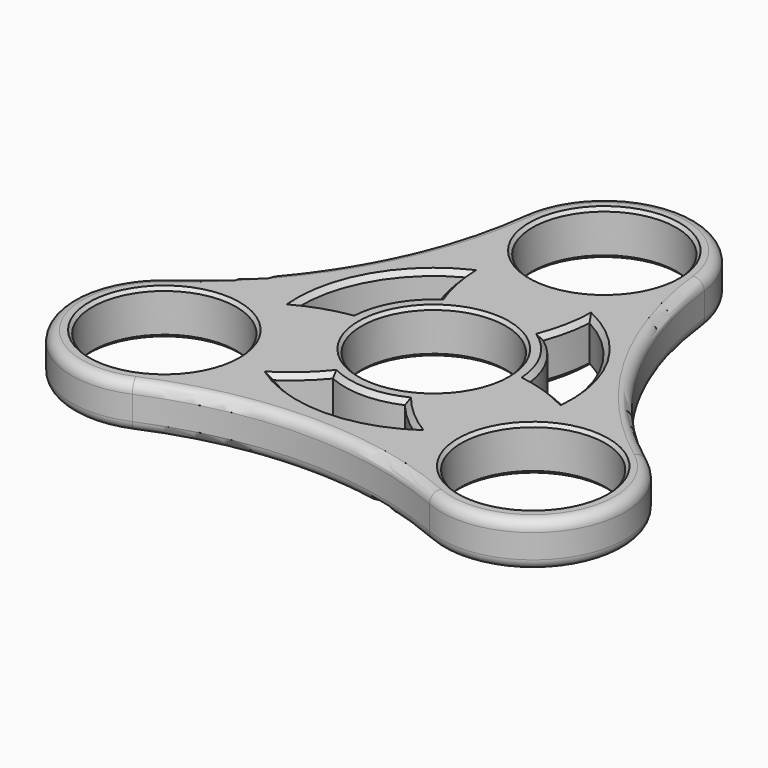
from build123d import *

# Parameters (mm, degrees)
F0_R          = 11.2522
F1_DEPTH      = 7
F2_R          = 11.2395
F3_DEPTH      = 7.001
F5_DEPTH      = 7.001
F6_R          = 1.625
F7_T3_ANGLE   = 75.0183506804
F7_S4_R       = 25.4
F7_T5_DEPTH   = 15
F7_S6_R       = 25.4
F7_T7_DEPTH   = 15
F7_T10_ANGLE  = 25.1712856634
F7_S11_R      = 13.843
F7_T12_DEPTH  = 7
F7_S13_R      = 20.701
F7_T14_DEPTH  = 7
F7_T17_ANGLE  = 63.8377846637
F7_S18_R      = 25.4
F7_T19_DEPTH  = 9
F7_S20_R      = 25.4
F7_T21_DEPTH  = 9
F7_T24_ANGLE  = 25.1712856634
F7_S25_R      = 13.843
F7_T26_DEPTH  = 7
F7_S27_R      = 20.701
F7_T28_DEPTH  = 7
F7_T31_ANGLE  = 25.1712856634
F7_S32_R      = 20.701
F7_T33_DEPTH  = 7
F7_S34_R      = 13.843
F7_T35_DEPTH  = 7
F7_T38_ANGLE  = 63.8377846637
F7_S39_R      = 25.4
F7_T40_DEPTH  = 9
F7_S41_R      = 25.4
F7_T42_DEPTH  = 9
F7_T45_ANGLE  = 25.1712856634
F7_S46_R      = 20.701
F7_T47_DEPTH  = 7
F7_S48_R      = 13.843
F7_T49_DEPTH  = 7
F7_T52_ANGLE  = 75.0183506804
F7_S53_R      = 25.4
F7_T54_DEPTH  = 15
F7_S55_R      = 25.4
F7_T56_DEPTH  = 15
F7_T59_ANGLE  = 25.1712856634
F7_S60_R      = 20.701
F7_T61_DEPTH  = 7
F7_S62_R      = 13.843
F7_T63_DEPTH  = 7
F7_T66_ANGLE  = 63.8377846637
F7_S67_R      = 25.4
F7_T68_DEPTH  = 9
F7_S69_R      = 25.4
F7_T70_DEPTH  = 9
F7_T73_ANGLE  = 25.1712856634
F7_S74_R      = 20.701
F7_T75_DEPTH  = 7
F7_S76_R      = 13.843
F7_T77_DEPTH  = 7
F7_T80_ANGLE  = 75.0183506804
F7_S81_R      = 25.4
F7_T82_DEPTH  = 15
F7_S83_R      = 25.4
F7_T84_DEPTH  = 15
F7_T87_ANGLE  = 75.0183506804
F7_S88_R      = 25.4
F7_T89_DEPTH  = 15
F7_S90_R      = 25.4
F7_T91_DEPTH  = 15
F7_T94_ANGLE  = 63.8377846637
F7_S95_R      = 25.4
F7_T96_DEPTH  = 9
F7_S97_R      = 25.4
F7_T98_DEPTH  = 9
F7_T101_ANGLE = 25.1712856634
F7_S102_R     = 20.701
F7_T103_DEPTH = 7
F7_S104_R     = 13.843
F7_T105_DEPTH = 7
F7_T108_ANGLE = 25.1712856634
F7_S109_R     = 20.701
F7_T110_DEPTH = 7
F7_S111_R     = 13.843
F7_T112_DEPTH = 7
F7_T115_ANGLE = 25.1712856634
F7_S116_R     = 20.701
F7_T117_DEPTH = 7
F7_S118_R     = 13.843
F7_T119_DEPTH = 7
F7_T122_ANGLE = 75.0183506804
F7_S123_R     = 25.4
F7_T124_DEPTH = 15
F7_S125_R     = 25.4
F7_T126_DEPTH = 15
F7_T129_ANGLE = 63.8377846637
F7_S130_R     = 25.4
F7_T131_DEPTH = 9
F7_S132_R     = 25.4
F7_T133_DEPTH = 9
F7_T136_ANGLE = 25.1712856634
F7_S137_R     = 20.701
F7_T138_DEPTH = 7
F7_S139_R     = 13.843
F7_T140_DEPTH = 7
F7_T143_ANGLE = 25.1712856634
F7_S144_R     = 13.843
F7_T145_DEPTH = 7
F7_S146_R     = 20.701
F7_T147_DEPTH = 7
F7_T150_ANGLE = 75.0183506804
F7_S151_R     = 25.4
F7_T152_DEPTH = 15
F7_S153_R     = 25.4
F7_T154_DEPTH = 15
F7_T157_ANGLE = 25.1712856634
F7_S158_R     = 13.843
F7_T159_DEPTH = 7
F7_S160_R     = 20.701
F7_T161_DEPTH = 7
F7_T164_ANGLE = 63.8377846637
F7_S165_R     = 25.4
F7_T166_DEPTH = 9
F7_S167_R     = 25.4
F7_T168_DEPTH = 9
F7_T172_ANGLE = 25.1712856634
F7_S173_R     = 20.701
F7_T174_DEPTH = 7
F7_T177_ANGLE = 75.0183506804
F7_S178_R     = 25.4
F7_T179_DEPTH = 15
F7_T184_ANGLE = 25.1712856634
F7_S185_R     = 20.701
F7_T186_DEPTH = 7
F7_T189_ANGLE = 75.0183506804
F7_S190_R     = 25.4
F7_T191_DEPTH = 15
F7_T196_ANGLE = 63.8377846637
F7_S197_R     = 25.4
F7_T198_DEPTH = 9
F7_T201_ANGLE = 25.1712856634
F7_S202_R     = 13.843
F7_T203_DEPTH = 7
F7_T208_ANGLE = 25.1712856634
F7_S209_R     = 13.843
F7_T210_DEPTH = 7
F7_T213_ANGLE = 63.8377846637
F7_S214_R     = 25.4
F7_T215_DEPTH = 9
F7_T220_ANGLE = 75.0183506804
F7_S221_R     = 25.4
F7_T222_DEPTH = 15
F7_T225_ANGLE = 25.1712856634
F7_S226_R     = 20.701
F7_T227_DEPTH = 7
F7_T232_ANGLE = 25.1712856634
F7_S233_R     = 13.843
F7_T234_DEPTH = 7
F7_T237_ANGLE = 63.8377846637
F7_S238_R     = 25.4
F7_T239_DEPTH = 9
F7_T244_ANGLE = 25.1712856634
F7_S245_R     = 13.843
F7_T246_DEPTH = 7
F7_T249_ANGLE = 63.8377846637
F7_S250_R     = 25.4
F7_T251_DEPTH = 9
F7_T256_ANGLE = 25.1712856634
F7_S257_R     = 20.701
F7_T258_DEPTH = 7
F7_T261_ANGLE = 75.0183506804
F7_S262_R     = 25.4
F7_T263_DEPTH = 15
F7_T268_ANGLE = 75.0183506804
F7_S269_R     = 25.4
F7_T270_DEPTH = 15
F7_T273_ANGLE = 25.1712856634
F7_S274_R     = 20.701
F7_T275_DEPTH = 7
F7_T280_ANGLE = 25.1712856634
F7_S281_R     = 13.843
F7_T282_DEPTH = 7
F7_T285_ANGLE = 63.8377846637
F7_S286_R     = 25.4
F7_T287_DEPTH = 9
F7_T292_ANGLE = 25.1712856634
F7_S293_R     = 13.843
F7_T294_DEPTH = 7
F7_T297_ANGLE = 63.8377846637
F7_S298_R     = 25.4
F7_T299_DEPTH = 9
F7_T304_ANGLE = 25.1712856634
F7_S305_R     = 20.701
F7_T306_DEPTH = 7
F7_T309_ANGLE = 75.0183506804
F7_S310_R     = 25.4
F7_T311_DEPTH = 15
F7_T316_ANGLE = 75.0183506804
F7_S317_R     = 25.4
F7_T318_DEPTH = 15
F7_T321_ANGLE = 25.1712856634
F7_S322_R     = 20.701
F7_T323_DEPTH = 7
F7_T328_ANGLE = 75.0183506804
F7_S329_R     = 25.4
F7_T330_DEPTH = 15
F7_T333_ANGLE = 25.1712856634
F7_S334_R     = 20.701
F7_T335_DEPTH = 7
F7_T340_ANGLE = 63.8377846637
F7_S341_R     = 25.4
F7_T342_DEPTH = 9
F7_T345_ANGLE = 25.1712856634
F7_S346_R     = 13.843
F7_T347_DEPTH = 7
F7_T352_ANGLE = 25.1712856634
F7_S353_R     = 13.843
F7_T354_DEPTH = 7
F7_T357_ANGLE = 63.8377846637
F7_S358_R     = 25.4
F7_T359_DEPTH = 9
F7_T364_ANGLE = 75.0183506804
F7_S365_R     = 25.4
F7_T366_DEPTH = 15
F7_T369_ANGLE = 25.1712856634
F7_S370_R     = 20.701
F7_T371_DEPTH = 7
F7_T376_ANGLE = 63.8377846637
F7_S377_R     = 25.4
F7_T378_DEPTH = 9
F7_T381_ANGLE = 25.1712856634
F7_S382_R     = 13.843
F7_T383_DEPTH = 7
F7_T388_ANGLE = 75.0183506804
F7_S389_R     = 25.4
F7_T390_DEPTH = 15
F7_T393_ANGLE = 25.1712856634
F7_S394_R     = 20.701
F7_T395_DEPTH = 7
F7_T400_ANGLE = 25.1712856634
F7_S401_R     = 13.843
F7_T402_DEPTH = 7
F7_T405_ANGLE = 63.8377846637
F7_S406_R     = 25.4
F7_T407_DEPTH = 9
F7_T412_ANGLE = 25.1712856634
F7_S413_R     = 20.701
F7_T414_DEPTH = 7
F7_T417_ANGLE = 75.0183506804
F7_S418_R     = 25.4
F7_T419_DEPTH = 15
F7_T424_ANGLE = 63.8377846637
F7_S425_R     = 25.4
F7_T426_DEPTH = 9
F7_T429_ANGLE = 25.1712856634
F7_S430_R     = 13.843
F7_T431_DEPTH = 7
F7_T436_ANGLE = 75.0183506804
F7_S437_R     = 25.4
F7_T438_DEPTH = 15
F7_T441_ANGLE = 25.1712856634
F7_S442_R     = 20.701
F7_T443_DEPTH = 7
F7_T448_ANGLE = 63.8377846637
F7_S449_R     = 25.4
F7_T450_DEPTH = 9
F7_T453_ANGLE = 25.1712856634
F7_S454_R     = 13.843
F7_T455_DEPTH = 7
F8_SIZE       = 0.5


# Not quite as in the source:
# - a fillet or chamfer that OpenCascade refuses, or shapes differently, is made with other operations: its cross-section is extruded or revolved along the edge and cut away or added


with BuildPart() as f1:
    # F0 (on Top) → F1 (new body)
    with BuildSketch(Plane.XY):
        with BuildLine():
            ThreePointArc((37.4145413955, -5.1495366448), (21.713132902, 12.5325990694), (14.2502695702, 34.9713562316))
            ThreePointArc((14.2502695702, 34.9713562316), (-0.0001243489, 47.6249999995), (-14.2502989826, 34.9711092792))
            ThreePointArc((-14.2502989826, 34.9711092792), (-21.7127734575, 12.5322227915), (-37.4138755234, -5.1501850199))
            ThreePointArc((-37.4138755234, -5.1501850199), (-41.2470555173, -23.8182100517), (-23.1633773799, -29.8322779327))
            ThreePointArc((-23.1633773799, -29.8322779327), (0.0005055885, -25.0755271592), (23.1644709862, -29.83187651))
            ThreePointArc((23.1644709862, -29.83187651), (41.2480448991, -23.8174952461), (37.4145413955, -5.1495366448))
        make_face()
        Circle(F0_R, mode=Mode.SUBTRACT)
    extrude(amount=F1_DEPTH)

    # F2 (on face) → F3 (cut, through all)
    with BuildSketch(Plane.XY.offset(7)):
        with Locations((0, 33.274)):
            Circle(F2_R)
        with Locations((-28.7836054376, -16.5806670429)):
            Circle(F2_R)
        with Locations((28.7836054376, -16.5806670429)):
            Circle(F2_R)
    extrude(amount=-F3_DEPTH, mode=Mode.SUBTRACT)

    # F4 (on face) → F5 (cut, through all)
    with BuildSketch(Plane.XY.offset(7)):
        with BuildLine():
            ThreePointArc((5.6160809719, -12.6525998718), (-6.831e-07, -13.843), (-5.6160822206, -12.6525993176))
            ThreePointArc((-5.6160822206, -12.6525993176), (-8.1436475782, -15.2823065658), (-11.021805406, -17.5228766643))
            ThreePointArc((-11.021805406, -17.5228766643), (-1.0215e-06, -20.701), (11.0218036767, -17.522877752))
            ThreePointArc((11.0218036767, -17.522877752), (8.14364607, -15.2823073695), (5.6160809719, -12.6525998718))
        make_face()
        with BuildLine():
            ThreePointArc((-8.1494313227, 11.1899695315), (-9.1630419253, 14.6937589651), (-9.6643536357, 18.3066018093))
            ThreePointArc((-9.6643536357, 18.3066018093), (-17.927591373, 10.3505008846), (-20.686159119, -0.7837231035))
            ThreePointArc((-20.686159119, -0.7837231035), (-17.3066894454, 0.5885493087), (-13.7655133989, 1.4626311446))
            ThreePointArc((-13.7655133989, 1.4626311446), (-11.9883893231, 6.9215005916), (-8.1494313227, 11.1899695315))
        make_face()
        with BuildLine():
            ThreePointArc((9.6643554423, 18.3066008556), (9.1630433754, 14.6937580608), (8.149432427, 11.1899687273))
            ThreePointArc((8.149432427, 11.1899687273), (11.9883900061, 6.9214994084), (13.7655135432, 1.4626297861))
            ThreePointArc((13.7655135432, 1.4626297861), (17.3066895035, 0.5885476007), (20.6861590417, -0.783725145))
            ThreePointArc((20.6861590417, -0.783725145), (17.9275923945, 10.3504991154), (9.6643554423, 18.3066008556))
        make_face()
    extrude(amount=-F5_DEPTH, mode=Mode.SUBTRACT)

    # F6
    f6_edges = [f1.edges().sort_by_distance(p)[0] for p in [
        (0.000506, -25.075527, 7),
        (0.000506, -25.075527, 0),
        (41.248045, -23.817495, 0),
        (41.248045, -23.817495, 7),
        (21.713133, 12.532599, 0),
        (21.713133, 12.532599, 7),
        (-41.247056, -23.81821, 0),
        (-0.000124, 47.625, 0),
        (-21.712773, 12.532223, 0),
        (-41.247056, -23.81821, 7),
        (-0.000124, 47.625, 7),
        (-21.712773, 12.532223, 7),
    ]]
    fillet(f6_edges, radius=F6_R)

    # F7: chamfer of 0.75 on 24 edges, made by hand


with BuildPart() as f7_tool1:
    # F7_s2 → F7_t3 (revolve)
    with BuildSketch(Plane(origin=(0, 0, 0), x_dir=(0, 0, 1), z_dir=(0.9239408224, 0.3825354319, 0))):
        Polygon((7, -21.451), (6.25, -20.701), (7, -20.701), align=None)
    revolve(axis=Axis((0, 0, 7), (0, 0, 1)), revolution_arc=F7_T3_ANGLE)

    # F7_s4 → F7_t5 (cut, symmetric)
    with BuildSketch(Plane.XY.offset(6.6)):
        with Locations((15.6803190028, 19.9821819622)):
            Circle(F7_S4_R)
    extrude(amount=F7_T5_DEPTH, both=True, mode=Mode.SUBTRACT)

    # F7_s6 → F7_t7 (cut, symmetric)
    with BuildSketch(Plane.XY.offset(6.6)):
        with Locations((-9.4649200271, -23.5706446429)):
            Circle(F7_S6_R)
    extrude(amount=F7_T7_DEPTH, both=True, mode=Mode.SUBTRACT)


with BuildPart() as f7_tool8:
    # F7_s9 → F7_t10 (revolve)
    with BuildSketch(Plane(origin=(-4.8460279311, 10.583246727, 0), x_dir=(0, 0, 1), z_dir=(0.4163261949, -0.9092153207, 0))):
        Polygon((7, 2.0741079466), (6.25, 2.8241079466), (7, 2.8241079466), align=None)
    revolve(axis=Axis((15.6803190028, 19.9821819622, 7), (0, 0, -1)), revolution_arc=F7_T10_ANGLE)

    # F7_s11 → F7_t12 (cut, symmetric)
    with BuildSketch(Plane.XY.offset(6.6)):
        Circle(F7_S11_R)
    extrude(amount=F7_T12_DEPTH, both=True, mode=Mode.SUBTRACT)

    # F7_s13 → F7_t14 (intersect, symmetric)
    with BuildSketch(Plane.XY.offset(6.6)):
        Circle(F7_S13_R)
    extrude(amount=F7_T14_DEPTH, both=True, mode=Mode.INTERSECT)


with BuildPart() as f7_tool15:
    # F7_s16 → F7_t17 (revolve)
    with BuildSketch(Plane(origin=(0, 0, 0), x_dir=(0, 0, 1), z_dir=(0.0334846794, -0.9994392309, 0))):
        Polygon((7, 13.093), (6.25, 13.843), (7, 13.843), align=None)
    revolve(axis=Axis((0, 0, 7), (0, 0, -1)), revolution_arc=F7_T17_ANGLE)

    # F7_s18 → F7_t19 (cut, symmetric)
    with BuildSketch(Plane.XY.offset(6.6)):
        with Locations((15.6803190028, 19.9821819622)):
            Circle(F7_S18_R)
    extrude(amount=F7_T19_DEPTH, both=True, mode=Mode.SUBTRACT)

    # F7_s20 → F7_t21 (cut, symmetric)
    with BuildSketch(Plane.XY.offset(6.6)):
        with Locations((-9.4649200271, -23.5706446429)):
            Circle(F7_S20_R)
    extrude(amount=F7_T21_DEPTH, both=True, mode=Mode.SUBTRACT)


with BuildPart() as f7_tool22:
    # F7_s23 → F7_t24 (revolve)
    with BuildSketch(Plane(origin=(-17.3382017848, -10.2408889637, 0), x_dir=(0, 0, 1), z_dir=(-0.8610224768, -0.5085669027, 0))):
        Polygon((7, 9.1686902329), (6.25, 9.9186902329), (7, 9.9186902329), align=None)
    revolve(axis=Axis((-9.4649200271, -23.5706446429, 7), (0, 0, -1)), revolution_arc=F7_T24_ANGLE)

    # F7_s25 → F7_t26 (cut, symmetric)
    with BuildSketch(Plane.XY.offset(6.6)):
        Circle(F7_S25_R)
    extrude(amount=F7_T26_DEPTH, both=True, mode=Mode.SUBTRACT)

    # F7_s27 → F7_t28 (intersect, symmetric)
    with BuildSketch(Plane.XY.offset(6.6)):
        Circle(F7_S27_R)
    extrude(amount=F7_T28_DEPTH, both=True, mode=Mode.INTERSECT)


with BuildPart() as f7_tool29:
    # F7_s30 → F7_t31 (revolve)
    with BuildSketch(Plane(origin=(-0.1997691075, 20.1357676834, 0), x_dir=(0, 0, 1), z_dir=(-0.0099206189, 0.9999507894, 0))):
        Polygon((7, 9.1686902329), (6.25, 9.9186902329), (7, 9.9186902329), align=None)
    revolve(axis=Axis((-15.6803170308, 19.9821835097, 7), (0, 0, -1)), revolution_arc=F7_T31_ANGLE)

    # F7_s32 → F7_t33 (intersect, symmetric)
    with BuildSketch(Plane.XY.offset(6.6)):
        Circle(F7_S32_R)
    extrude(amount=F7_T33_DEPTH, both=True, mode=Mode.INTERSECT)

    # F7_s34 → F7_t35 (cut, symmetric)
    with BuildSketch(Plane.XY.offset(6.6)):
        Circle(F7_S34_R)
    extrude(amount=F7_T35_DEPTH, both=True, mode=Mode.SUBTRACT)


with BuildPart() as f7_tool36:
    # F7_s37 → F7_t38 (revolve)
    with BuildSketch(Plane(origin=(0, 0, 0), x_dir=(0, 0, 1), z_dir=(-0.8822821032, 0.4707210325, 0))):
        Polygon((7, 13.093), (6.25, 13.843), (7, 13.843), align=None)
    revolve(axis=Axis((0, 0, 7), (0, 0, -1)), revolution_arc=F7_T38_ANGLE)

    # F7_s39 → F7_t40 (cut, symmetric)
    with BuildSketch(Plane.XY.offset(6.6)):
        with Locations((-15.6803170308, 19.9821835097)):
            Circle(F7_S39_R)
    extrude(amount=F7_T40_DEPTH, both=True, mode=Mode.SUBTRACT)

    # F7_s41 → F7_t42 (cut, symmetric)
    with BuildSketch(Plane.XY.offset(6.6)):
        with Locations((9.4649177009, -23.570645577)):
            Circle(F7_S41_R)
    extrude(amount=F7_T42_DEPTH, both=True, mode=Mode.SUBTRACT)


with BuildPart() as f7_tool43:
    # F7_s44 → F7_t45 (revolve)
    with BuildSketch(Plane(origin=(11.5883744856, -1.0948400677, 0), x_dir=(0, 0, 1), z_dir=(-0.9955666627, 0.0940585993, 0))):
        Polygon((7, 2.0741079466), (6.25, 2.8241079466), (7, 2.8241079466), align=None)
    revolve(axis=Axis((9.4649177009, -23.570645577, 7), (0, 0, -1)), revolution_arc=F7_T45_ANGLE)

    # F7_s46 → F7_t47 (intersect, symmetric)
    with BuildSketch(Plane.XY.offset(6.6)):
        Circle(F7_S46_R)
    extrude(amount=F7_T47_DEPTH, both=True, mode=Mode.INTERSECT)

    # F7_s48 → F7_t49 (cut, symmetric)
    with BuildSketch(Plane.XY.offset(6.6)):
        Circle(F7_S48_R)
    extrude(amount=F7_T49_DEPTH, both=True, mode=Mode.SUBTRACT)


with BuildPart() as f7_tool50:
    # F7_s51 → F7_t52 (revolve)
    with BuildSketch(Plane(origin=(0, 0, 0), x_dir=(0, 0, 1), z_dir=(-0.1306850093, -0.9914239398, 0))):
        Polygon((7, -21.451), (6.25, -20.701), (7, -20.701), align=None)
    revolve(axis=Axis((0, 0, 7), (0, 0, 1)), revolution_arc=F7_T52_ANGLE)

    # F7_s53 → F7_t54 (cut, symmetric)
    with BuildSketch(Plane.XY.offset(6.6)):
        with Locations((-15.6803170308, 19.9821835097)):
            Circle(F7_S53_R)
    extrude(amount=F7_T54_DEPTH, both=True, mode=Mode.SUBTRACT)

    # F7_s55 → F7_t56 (cut, symmetric)
    with BuildSketch(Plane.XY.offset(6.6)):
        with Locations((9.4649177009, -23.570645577)):
            Circle(F7_S55_R)
    extrude(amount=F7_T56_DEPTH, both=True, mode=Mode.SUBTRACT)


with BuildPart() as f7_tool57:
    # F7_s58 → F7_t59 (revolve)
    with BuildSketch(Plane(origin=(17.5379708923, -9.8948787197, 0), x_dir=(0, 0, 1), z_dir=(0.8709430956, -0.4913838868, 0))):
        Polygon((7, 9.1686902329), (6.25, 9.9186902329), (7, 9.9186902329), align=None)
    revolve(axis=Axis((25.1452370578, 3.5884611332, 7), (0, 0, -1)), revolution_arc=F7_T59_ANGLE)

    # F7_s60 → F7_t61 (intersect, symmetric)
    with BuildSketch(Plane.XY.offset(6.6)):
        Circle(F7_S60_R)
    extrude(amount=F7_T61_DEPTH, both=True, mode=Mode.INTERSECT)

    # F7_s62 → F7_t63 (cut, symmetric)
    with BuildSketch(Plane.XY.offset(6.6)):
        Circle(F7_S62_R)
    extrude(amount=F7_T63_DEPTH, both=True, mode=Mode.SUBTRACT)


with BuildPart() as f7_tool64:
    # F7_s65 → F7_t66 (revolve)
    with BuildSketch(Plane(origin=(0, 0, 0), x_dir=(0, 0, 1), z_dir=(0.8487974238, 0.5287181984, 0))):
        Polygon((7, 13.093), (6.25, 13.843), (7, 13.843), align=None)
    revolve(axis=Axis((0, 0, 7), (0, 0, -1)), revolution_arc=F7_T66_ANGLE)

    # F7_s67 → F7_t68 (cut, symmetric)
    with BuildSketch(Plane.XY.offset(6.6)):
        with Locations((25.1452370578, 3.5884611332)):
            Circle(F7_S67_R)
    extrude(amount=F7_T68_DEPTH, both=True, mode=Mode.SUBTRACT)

    # F7_s69 → F7_t70 (cut, symmetric)
    with BuildSketch(Plane.XY.offset(6.6)):
        with Locations((-25.1452367037, 3.5884636148)):
            Circle(F7_S69_R)
    extrude(amount=F7_T70_DEPTH, both=True, mode=Mode.SUBTRACT)


with BuildPart() as f7_tool71:
    # F7_s72 → F7_t73 (revolve)
    with BuildSketch(Plane(origin=(-6.7423465545, -9.4884066593, 0), x_dir=(0, 0, 1), z_dir=(0.5792404678, 0.8151567214, 0))):
        Polygon((7, 2.0741079466), (6.25, 2.8241079466), (7, 2.8241079466), align=None)
    revolve(axis=Axis((-25.1452367037, 3.5884636148, 7), (0, 0, -1)), revolution_arc=F7_T73_ANGLE)

    # F7_s74 → F7_t75 (intersect, symmetric)
    with BuildSketch(Plane.XY.offset(6.6)):
        Circle(F7_S74_R)
    extrude(amount=F7_T75_DEPTH, both=True, mode=Mode.INTERSECT)

    # F7_s76 → F7_t77 (cut, symmetric)
    with BuildSketch(Plane.XY.offset(6.6)):
        Circle(F7_S76_R)
    extrude(amount=F7_T77_DEPTH, both=True, mode=Mode.SUBTRACT)


with BuildPart() as f7_tool78:
    # F7_s79 → F7_t80 (revolve)
    with BuildSketch(Plane(origin=(0, 0, 0), x_dir=(0, 0, 1), z_dir=(-0.7932558131, 0.6088885079, 0))):
        Polygon((7, -21.451), (6.25, -20.701), (7, -20.701), align=None)
    revolve(axis=Axis((0, 0, 7), (0, 0, 1)), revolution_arc=F7_T80_ANGLE)

    # F7_s81 → F7_t82 (cut, symmetric)
    with BuildSketch(Plane.XY.offset(6.6)):
        with Locations((25.1452370578, 3.5884611332)):
            Circle(F7_S81_R)
    extrude(amount=F7_T82_DEPTH, both=True, mode=Mode.SUBTRACT)

    # F7_s83 → F7_t84 (cut, symmetric)
    with BuildSketch(Plane.XY.offset(6.6)):
        with Locations((-25.1452367037, 3.5884636148)):
            Circle(F7_S83_R)
    extrude(amount=F7_T84_DEPTH, both=True, mode=Mode.SUBTRACT)


with BuildPart() as f7_tool85:
    # F7_s86 → F7_t87 (revolve)
    with BuildSketch(Plane(origin=(0, 0, 0), x_dir=(0, 0, 1), z_dir=(-0.7932558131, 0.6088885079, 0))):
        Polygon((0, -21.451), (0.75, -20.701), (0, -20.701), align=None)
    revolve(axis=Axis((0, 0, 0), (0, 0, 1)), revolution_arc=F7_T87_ANGLE)

    # F7_s88 → F7_t89 (cut, symmetric)
    with BuildSketch(Plane.XY.offset(0.4)):
        with Locations((25.1452370578, 3.5884611332)):
            Circle(F7_S88_R)
    extrude(amount=F7_T89_DEPTH, both=True, mode=Mode.SUBTRACT)

    # F7_s90 → F7_t91 (cut, symmetric)
    with BuildSketch(Plane.XY.offset(0.4)):
        with Locations((-25.1452367037, 3.5884636148)):
            Circle(F7_S90_R)
    extrude(amount=F7_T91_DEPTH, both=True, mode=Mode.SUBTRACT)


with BuildPart() as f7_tool92:
    # F7_s93 → F7_t94 (revolve)
    with BuildSketch(Plane(origin=(0, 0, 0), x_dir=(0, 0, 1), z_dir=(-0.8487973716, 0.5287182822, 0))):
        Polygon((0, -13.093), (0.75, -13.843), (0, -13.843), align=None)
    revolve(axis=Axis((0, 0, 0), (0, 0, 1)), revolution_arc=F7_T94_ANGLE)

    # F7_s95 → F7_t96 (cut, symmetric)
    with BuildSketch(Plane.XY.offset(0.4)):
        with Locations((25.1452370578, 3.5884611332)):
            Circle(F7_S95_R)
    extrude(amount=F7_T96_DEPTH, both=True, mode=Mode.SUBTRACT)

    # F7_s97 → F7_t98 (cut, symmetric)
    with BuildSketch(Plane.XY.offset(0.4)):
        with Locations((-25.1452367037, 3.5884636148)):
            Circle(F7_S97_R)
    extrude(amount=F7_T98_DEPTH, both=True, mode=Mode.SUBTRACT)


with BuildPart() as f7_tool99:
    # F7_s100 → F7_t101 (revolve)
    with BuildSketch(Plane(origin=(-17.5379718688, -9.8948769889, 0), x_dir=(0, 0, 1), z_dir=(-0.8709431441, -0.4913838008, 0))):
        Polygon((0, -9.1686902329), (0.75, -9.9186902329), (0, -9.9186902329), align=None)
    revolve(axis=Axis((-25.1452367037, 3.5884636148, 0), (0, 0, 1)), revolution_arc=F7_T101_ANGLE)

    # F7_s102 → F7_t103 (intersect, symmetric)
    with BuildSketch(Plane.XY.offset(0.4)):
        Circle(F7_S102_R)
    extrude(amount=F7_T103_DEPTH, both=True, mode=Mode.INTERSECT)

    # F7_s104 → F7_t105 (cut, symmetric)
    with BuildSketch(Plane.XY.offset(0.4)):
        Circle(F7_S104_R)
    extrude(amount=F7_T105_DEPTH, both=True, mode=Mode.SUBTRACT)


with BuildPart() as f7_tool106:
    # F7_s107 → F7_t108 (revolve)
    with BuildSketch(Plane(origin=(6.7423456181, -9.4884073247, 0), x_dir=(0, 0, 1), z_dir=(-0.5792403874, 0.8151567786, 0))):
        Polygon((0, -2.0741079466), (0.75, -2.8241079466), (0, -2.8241079466), align=None)
    revolve(axis=Axis((25.1452370578, 3.5884611332, 0), (0, 0, 1)), revolution_arc=F7_T108_ANGLE)

    # F7_s109 → F7_t110 (intersect, symmetric)
    with BuildSketch(Plane.XY.offset(0.4)):
        Circle(F7_S109_R)
    extrude(amount=F7_T110_DEPTH, both=True, mode=Mode.INTERSECT)

    # F7_s111 → F7_t112 (cut, symmetric)
    with BuildSketch(Plane.XY.offset(0.4)):
        Circle(F7_S111_R)
    extrude(amount=F7_T112_DEPTH, both=True, mode=Mode.SUBTRACT)


with BuildPart() as f7_tool113:
    # F7_s114 → F7_t115 (revolve)
    with BuildSketch(Plane(origin=(17.3382007741, -10.2408906747, 0), x_dir=(0, 0, 1), z_dir=(0.8610224266, -0.5085669877, 0))):
        Polygon((0, -9.1686902329), (0.75, -9.9186902329), (0, -9.9186902329), align=None)
    revolve(axis=Axis((9.4649177009, -23.570645577, 0), (0, 0, 1)), revolution_arc=F7_T115_ANGLE)

    # F7_s116 → F7_t117 (intersect, symmetric)
    with BuildSketch(Plane.XY.offset(0.4)):
        Circle(F7_S116_R)
    extrude(amount=F7_T117_DEPTH, both=True, mode=Mode.INTERSECT)

    # F7_s118 → F7_t119 (cut, symmetric)
    with BuildSketch(Plane.XY.offset(0.4)):
        Circle(F7_S118_R)
    extrude(amount=F7_T119_DEPTH, both=True, mode=Mode.SUBTRACT)


with BuildPart() as f7_tool120:
    # F7_s121 → F7_t122 (revolve)
    with BuildSketch(Plane(origin=(0, 0, 0), x_dir=(0, 0, 1), z_dir=(-0.1306850093, -0.9914239398, 0))):
        Polygon((0, -21.451), (0.75, -20.701), (0, -20.701), align=None)
    revolve(axis=Axis((0, 0, 0), (0, 0, 1)), revolution_arc=F7_T122_ANGLE)

    # F7_s123 → F7_t124 (cut, symmetric)
    with BuildSketch(Plane.XY.offset(0.4)):
        with Locations((-15.6803170308, 19.9821835097)):
            Circle(F7_S123_R)
    extrude(amount=F7_T124_DEPTH, both=True, mode=Mode.SUBTRACT)

    # F7_s125 → F7_t126 (cut, symmetric)
    with BuildSketch(Plane.XY.offset(0.4)):
        with Locations((9.4649177009, -23.570645577)):
            Circle(F7_S125_R)
    extrude(amount=F7_T126_DEPTH, both=True, mode=Mode.SUBTRACT)


with BuildPart() as f7_tool127:
    # F7_s128 → F7_t129 (revolve)
    with BuildSketch(Plane(origin=(0, 0, 0), x_dir=(0, 0, 1), z_dir=(-0.033484778, -0.9994392276, 0))):
        Polygon((0, -13.093), (0.75, -13.843), (0, -13.843), align=None)
    revolve(axis=Axis((0, 0, 0), (0, 0, 1)), revolution_arc=F7_T129_ANGLE)

    # F7_s130 → F7_t131 (cut, symmetric)
    with BuildSketch(Plane.XY.offset(0.4)):
        with Locations((-15.6803170308, 19.9821835097)):
            Circle(F7_S130_R)
    extrude(amount=F7_T131_DEPTH, both=True, mode=Mode.SUBTRACT)

    # F7_s132 → F7_t133 (cut, symmetric)
    with BuildSketch(Plane.XY.offset(0.4)):
        with Locations((9.4649177009, -23.570645577)):
            Circle(F7_S132_R)
    extrude(amount=F7_T133_DEPTH, both=True, mode=Mode.SUBTRACT)


with BuildPart() as f7_tool134:
    # F7_s135 → F7_t136 (revolve)
    with BuildSketch(Plane(origin=(4.8460289755, 10.5832462487, 0), x_dir=(0, 0, 1), z_dir=(-0.4163262846, -0.9092152796, 0))):
        Polygon((0, -2.0741079466), (0.75, -2.8241079466), (0, -2.8241079466), align=None)
    revolve(axis=Axis((-15.6803170308, 19.9821835097, 0), (0, 0, 1)), revolution_arc=F7_T136_ANGLE)

    # F7_s137 → F7_t138 (intersect, symmetric)
    with BuildSketch(Plane.XY.offset(0.4)):
        Circle(F7_S137_R)
    extrude(amount=F7_T138_DEPTH, both=True, mode=Mode.INTERSECT)

    # F7_s139 → F7_t140 (cut, symmetric)
    with BuildSketch(Plane.XY.offset(0.4)):
        Circle(F7_S139_R)
    extrude(amount=F7_T140_DEPTH, both=True, mode=Mode.SUBTRACT)


with BuildPart() as f7_tool141:
    # F7_s142 → F7_t143 (revolve)
    with BuildSketch(Plane(origin=(0.1997710946, 20.1357676637, 0), x_dir=(0, 0, 1), z_dir=(0.0099207175, 0.9999507885, 0))):
        Polygon((0, -9.1686902329), (0.75, -9.9186902329), (0, -9.9186902329), align=None)
    revolve(axis=Axis((15.6803190028, 19.9821819622, 0), (0, 0, 1)), revolution_arc=F7_T143_ANGLE)

    # F7_s144 → F7_t145 (cut, symmetric)
    with BuildSketch(Plane.XY.offset(0.4)):
        Circle(F7_S144_R)
    extrude(amount=F7_T145_DEPTH, both=True, mode=Mode.SUBTRACT)

    # F7_s146 → F7_t147 (intersect, symmetric)
    with BuildSketch(Plane.XY.offset(0.4)):
        Circle(F7_S146_R)
    extrude(amount=F7_T147_DEPTH, both=True, mode=Mode.INTERSECT)


with BuildPart() as f7_tool148:
    # F7_s149 → F7_t150 (revolve)
    with BuildSketch(Plane(origin=(0, 0, 0), x_dir=(0, 0, 1), z_dir=(0.9239408224, 0.3825354319, 0))):
        Polygon((0, -21.451), (0.75, -20.701), (0, -20.701), align=None)
    revolve(axis=Axis((0, 0, 0), (0, 0, 1)), revolution_arc=F7_T150_ANGLE)

    # F7_s151 → F7_t152 (cut, symmetric)
    with BuildSketch(Plane.XY.offset(0.4)):
        with Locations((15.6803190028, 19.9821819622)):
            Circle(F7_S151_R)
    extrude(amount=F7_T152_DEPTH, both=True, mode=Mode.SUBTRACT)

    # F7_s153 → F7_t154 (cut, symmetric)
    with BuildSketch(Plane.XY.offset(0.4)):
        with Locations((-9.4649200271, -23.5706446429)):
            Circle(F7_S153_R)
    extrude(amount=F7_T154_DEPTH, both=True, mode=Mode.SUBTRACT)


with BuildPart() as f7_tool155:
    # F7_s156 → F7_t157 (revolve)
    with BuildSketch(Plane(origin=(-11.5883745937, -1.0948389241, 0), x_dir=(0, 0, 1), z_dir=(0.995566672, 0.0940585011, 0))):
        Polygon((0, -2.0741079466), (0.75, -2.8241079466), (0, -2.8241079466), align=None)
    revolve(axis=Axis((-9.4649200271, -23.5706446429, 0), (0, 0, 1)), revolution_arc=F7_T157_ANGLE)

    # F7_s158 → F7_t159 (cut, symmetric)
    with BuildSketch(Plane.XY.offset(0.4)):
        Circle(F7_S158_R)
    extrude(amount=F7_T159_DEPTH, both=True, mode=Mode.SUBTRACT)

    # F7_s160 → F7_t161 (intersect, symmetric)
    with BuildSketch(Plane.XY.offset(0.4)):
        Circle(F7_S160_R)
    extrude(amount=F7_T161_DEPTH, both=True, mode=Mode.INTERSECT)


with BuildPart() as f7_tool162:
    # F7_s163 → F7_t164 (revolve)
    with BuildSketch(Plane(origin=(0, 0, 0), x_dir=(0, 0, 1), z_dir=(0.8822821496, 0.4707209454, 0))):
        Polygon((0, -13.093), (0.75, -13.843), (0, -13.843), align=None)
    revolve(axis=Axis((0, 0, 0), (0, 0, 1)), revolution_arc=F7_T164_ANGLE)

    # F7_s165 → F7_t166 (cut, symmetric)
    with BuildSketch(Plane.XY.offset(0.4)):
        with Locations((15.6803190028, 19.9821819622)):
            Circle(F7_S165_R)
    extrude(amount=F7_T166_DEPTH, both=True, mode=Mode.SUBTRACT)

    # F7_s167 → F7_t168 (cut, symmetric)
    with BuildSketch(Plane.XY.offset(0.4)):
        with Locations((-9.4649200271, -23.5706446429)):
            Circle(F7_S167_R)
    extrude(amount=F7_T168_DEPTH, both=True, mode=Mode.SUBTRACT)


with BuildPart() as f7_tool170:
    # F7_s171 → F7_t172 (revolve)
    with BuildSketch(Plane(origin=(-4.8460279311, 10.583246727, 0), x_dir=(0, 0, 1), z_dir=(0.4163261949, -0.9092153207, 0))):
        Polygon((7, 2.0741079466), (6.25, 2.8241079466), (7, 2.8241079466), align=None)
    revolve(axis=Axis((15.6803190028, 19.9821819622, 7), (0, 0, -1)), revolution_arc=F7_T172_ANGLE)

    # F7_s173 → F7_t174 (cut, symmetric)
    with BuildSketch(Plane.XY.offset(6.6)):
        Circle(F7_S173_R)
    extrude(amount=F7_T174_DEPTH, both=True, mode=Mode.SUBTRACT)


with BuildPart() as f7_tool175:
    # F7_s176 → F7_t177 (revolve)
    with BuildSketch(Plane(origin=(0, 0, 0), x_dir=(0, 0, 1), z_dir=(0.9239408224, 0.3825354319, 0))):
        Polygon((7, -21.451), (6.25, -20.701), (7, -20.701), align=None)
    revolve(axis=Axis((0, 0, 7), (0, 0, 1)), revolution_arc=F7_T177_ANGLE)

    # F7_s178 → F7_t179 (intersect, symmetric)
    with BuildSketch(Plane.XY.offset(6.6)):
        with Locations((15.6803190028, 19.9821819622)):
            Circle(F7_S178_R)
    extrude(amount=F7_T179_DEPTH, both=True, mode=Mode.INTERSECT)


with BuildPart() as f7_tool170_1:
    add(f7_tool170.part)

    # F7_t180: intersect F7_tool175
    add(f7_tool175.part, mode=Mode.INTERSECT)


with BuildPart() as f7_tool182:
    # F7_s183 → F7_t184 (revolve)
    with BuildSketch(Plane(origin=(-17.3382017848, -10.2408889637, 0), x_dir=(0, 0, 1), z_dir=(-0.8610224768, -0.5085669027, 0))):
        Polygon((7, 9.1686902329), (6.25, 9.9186902329), (7, 9.9186902329), align=None)
    revolve(axis=Axis((-9.4649200271, -23.5706446429, 7), (0, 0, -1)), revolution_arc=F7_T184_ANGLE)

    # F7_s185 → F7_t186 (cut, symmetric)
    with BuildSketch(Plane.XY.offset(6.6)):
        Circle(F7_S185_R)
    extrude(amount=F7_T186_DEPTH, both=True, mode=Mode.SUBTRACT)


with BuildPart() as f7_tool187:
    # F7_s188 → F7_t189 (revolve)
    with BuildSketch(Plane(origin=(0, 0, 0), x_dir=(0, 0, 1), z_dir=(0.9239408224, 0.3825354319, 0))):
        Polygon((7, -21.451), (6.25, -20.701), (7, -20.701), align=None)
    revolve(axis=Axis((0, 0, 7), (0, 0, 1)), revolution_arc=F7_T189_ANGLE)

    # F7_s190 → F7_t191 (intersect, symmetric)
    with BuildSketch(Plane.XY.offset(6.6)):
        with Locations((-9.4649200271, -23.5706446429)):
            Circle(F7_S190_R)
    extrude(amount=F7_T191_DEPTH, both=True, mode=Mode.INTERSECT)


with BuildPart() as f7_tool182_1:
    add(f7_tool182.part)

    # F7_t192: intersect F7_tool187
    add(f7_tool187.part, mode=Mode.INTERSECT)


with BuildPart() as f7_tool194:
    # F7_s195 → F7_t196 (revolve)
    with BuildSketch(Plane(origin=(0, 0, 0), x_dir=(0, 0, 1), z_dir=(0.0334846794, -0.9994392309, 0))):
        Polygon((7, 13.093), (6.25, 13.843), (7, 13.843), align=None)
    revolve(axis=Axis((0, 0, 7), (0, 0, -1)), revolution_arc=F7_T196_ANGLE)

    # F7_s197 → F7_t198 (intersect, symmetric)
    with BuildSketch(Plane.XY.offset(6.6)):
        with Locations((15.6803190028, 19.9821819622)):
            Circle(F7_S197_R)
    extrude(amount=F7_T198_DEPTH, both=True, mode=Mode.INTERSECT)


with BuildPart() as f7_tool199:
    # F7_s200 → F7_t201 (revolve)
    with BuildSketch(Plane(origin=(-4.8460279311, 10.583246727, 0), x_dir=(0, 0, 1), z_dir=(0.4163261949, -0.9092153207, 0))):
        Polygon((7, 2.0741079466), (6.25, 2.8241079466), (7, 2.8241079466), align=None)
    revolve(axis=Axis((15.6803190028, 19.9821819622, 7), (0, 0, -1)), revolution_arc=F7_T201_ANGLE)

    # F7_s202 → F7_t203 (intersect, symmetric)
    with BuildSketch(Plane.XY.offset(6.6)):
        Circle(F7_S202_R)
    extrude(amount=F7_T203_DEPTH, both=True, mode=Mode.INTERSECT)


with BuildPart() as f7_tool194_1:
    add(f7_tool194.part)

    # F7_t204: intersect F7_tool199
    add(f7_tool199.part, mode=Mode.INTERSECT)


with BuildPart() as f7_tool206:
    # F7_s207 → F7_t208 (revolve)
    with BuildSketch(Plane(origin=(-17.3382017848, -10.2408889637, 0), x_dir=(0, 0, 1), z_dir=(-0.8610224768, -0.5085669027, 0))):
        Polygon((7, 9.1686902329), (6.25, 9.9186902329), (7, 9.9186902329), align=None)
    revolve(axis=Axis((-9.4649200271, -23.5706446429, 7), (0, 0, -1)), revolution_arc=F7_T208_ANGLE)

    # F7_s209 → F7_t210 (intersect, symmetric)
    with BuildSketch(Plane.XY.offset(6.6)):
        Circle(F7_S209_R)
    extrude(amount=F7_T210_DEPTH, both=True, mode=Mode.INTERSECT)


with BuildPart() as f7_tool211:
    # F7_s212 → F7_t213 (revolve)
    with BuildSketch(Plane(origin=(0, 0, 0), x_dir=(0, 0, 1), z_dir=(0.0334846794, -0.9994392309, 0))):
        Polygon((7, 13.093), (6.25, 13.843), (7, 13.843), align=None)
    revolve(axis=Axis((0, 0, 7), (0, 0, -1)), revolution_arc=F7_T213_ANGLE)

    # F7_s214 → F7_t215 (intersect, symmetric)
    with BuildSketch(Plane.XY.offset(6.6)):
        with Locations((-9.4649200271, -23.5706446429)):
            Circle(F7_S214_R)
    extrude(amount=F7_T215_DEPTH, both=True, mode=Mode.INTERSECT)


with BuildPart() as f7_tool206_1:
    add(f7_tool206.part)

    # F7_t216: intersect F7_tool211
    add(f7_tool211.part, mode=Mode.INTERSECT)


with BuildPart() as f7_tool218:
    # F7_s219 → F7_t220 (revolve)
    with BuildSketch(Plane(origin=(0, 0, 0), x_dir=(0, 0, 1), z_dir=(-0.1306850093, -0.9914239398, 0))):
        Polygon((7, -21.451), (6.25, -20.701), (7, -20.701), align=None)
    revolve(axis=Axis((0, 0, 7), (0, 0, 1)), revolution_arc=F7_T220_ANGLE)

    # F7_s221 → F7_t222 (intersect, symmetric)
    with BuildSketch(Plane.XY.offset(6.6)):
        with Locations((-15.6803170308, 19.9821835097)):
            Circle(F7_S221_R)
    extrude(amount=F7_T222_DEPTH, both=True, mode=Mode.INTERSECT)


with BuildPart() as f7_tool223:
    # F7_s224 → F7_t225 (revolve)
    with BuildSketch(Plane(origin=(-0.1997691075, 20.1357676834, 0), x_dir=(0, 0, 1), z_dir=(-0.0099206189, 0.9999507894, 0))):
        Polygon((7, 9.1686902329), (6.25, 9.9186902329), (7, 9.9186902329), align=None)
    revolve(axis=Axis((-15.6803170308, 19.9821835097, 7), (0, 0, -1)), revolution_arc=F7_T225_ANGLE)

    # F7_s226 → F7_t227 (cut, symmetric)
    with BuildSketch(Plane.XY.offset(6.6)):
        Circle(F7_S226_R)
    extrude(amount=F7_T227_DEPTH, both=True, mode=Mode.SUBTRACT)


with BuildPart() as f7_tool218_1:
    add(f7_tool218.part)

    # F7_t228: intersect F7_tool223
    add(f7_tool223.part, mode=Mode.INTERSECT)


with BuildPart() as f7_tool230:
    # F7_s231 → F7_t232 (revolve)
    with BuildSketch(Plane(origin=(-0.1997691075, 20.1357676834, 0), x_dir=(0, 0, 1), z_dir=(-0.0099206189, 0.9999507894, 0))):
        Polygon((7, 9.1686902329), (6.25, 9.9186902329), (7, 9.9186902329), align=None)
    revolve(axis=Axis((-15.6803170308, 19.9821835097, 7), (0, 0, -1)), revolution_arc=F7_T232_ANGLE)

    # F7_s233 → F7_t234 (intersect, symmetric)
    with BuildSketch(Plane.XY.offset(6.6)):
        Circle(F7_S233_R)
    extrude(amount=F7_T234_DEPTH, both=True, mode=Mode.INTERSECT)


with BuildPart() as f7_tool235:
    # F7_s236 → F7_t237 (revolve)
    with BuildSketch(Plane(origin=(0, 0, 0), x_dir=(0, 0, 1), z_dir=(-0.8822821032, 0.4707210325, 0))):
        Polygon((7, 13.093), (6.25, 13.843), (7, 13.843), align=None)
    revolve(axis=Axis((0, 0, 7), (0, 0, -1)), revolution_arc=F7_T237_ANGLE)

    # F7_s238 → F7_t239 (intersect, symmetric)
    with BuildSketch(Plane.XY.offset(6.6)):
        with Locations((-15.6803170308, 19.9821835097)):
            Circle(F7_S238_R)
    extrude(amount=F7_T239_DEPTH, both=True, mode=Mode.INTERSECT)


with BuildPart() as f7_tool230_1:
    add(f7_tool230.part)

    # F7_t240: intersect F7_tool235
    add(f7_tool235.part, mode=Mode.INTERSECT)


with BuildPart() as f7_tool242:
    # F7_s243 → F7_t244 (revolve)
    with BuildSketch(Plane(origin=(11.5883744856, -1.0948400677, 0), x_dir=(0, 0, 1), z_dir=(-0.9955666627, 0.0940585993, 0))):
        Polygon((7, 2.0741079466), (6.25, 2.8241079466), (7, 2.8241079466), align=None)
    revolve(axis=Axis((9.4649177009, -23.570645577, 7), (0, 0, -1)), revolution_arc=F7_T244_ANGLE)

    # F7_s245 → F7_t246 (intersect, symmetric)
    with BuildSketch(Plane.XY.offset(6.6)):
        Circle(F7_S245_R)
    extrude(amount=F7_T246_DEPTH, both=True, mode=Mode.INTERSECT)


with BuildPart() as f7_tool247:
    # F7_s248 → F7_t249 (revolve)
    with BuildSketch(Plane(origin=(0, 0, 0), x_dir=(0, 0, 1), z_dir=(-0.8822821032, 0.4707210325, 0))):
        Polygon((7, 13.093), (6.25, 13.843), (7, 13.843), align=None)
    revolve(axis=Axis((0, 0, 7), (0, 0, -1)), revolution_arc=F7_T249_ANGLE)

    # F7_s250 → F7_t251 (intersect, symmetric)
    with BuildSketch(Plane.XY.offset(6.6)):
        with Locations((9.4649177009, -23.570645577)):
            Circle(F7_S250_R)
    extrude(amount=F7_T251_DEPTH, both=True, mode=Mode.INTERSECT)


with BuildPart() as f7_tool242_1:
    add(f7_tool242.part)

    # F7_t252: intersect F7_tool247
    add(f7_tool247.part, mode=Mode.INTERSECT)


with BuildPart() as f7_tool254:
    # F7_s255 → F7_t256 (revolve)
    with BuildSketch(Plane(origin=(11.5883744856, -1.0948400677, 0), x_dir=(0, 0, 1), z_dir=(-0.9955666627, 0.0940585993, 0))):
        Polygon((7, 2.0741079466), (6.25, 2.8241079466), (7, 2.8241079466), align=None)
    revolve(axis=Axis((9.4649177009, -23.570645577, 7), (0, 0, -1)), revolution_arc=F7_T256_ANGLE)

    # F7_s257 → F7_t258 (cut, symmetric)
    with BuildSketch(Plane.XY.offset(6.6)):
        Circle(F7_S257_R)
    extrude(amount=F7_T258_DEPTH, both=True, mode=Mode.SUBTRACT)


with BuildPart() as f7_tool259:
    # F7_s260 → F7_t261 (revolve)
    with BuildSketch(Plane(origin=(0, 0, 0), x_dir=(0, 0, 1), z_dir=(-0.1306850093, -0.9914239398, 0))):
        Polygon((7, -21.451), (6.25, -20.701), (7, -20.701), align=None)
    revolve(axis=Axis((0, 0, 7), (0, 0, 1)), revolution_arc=F7_T261_ANGLE)

    # F7_s262 → F7_t263 (intersect, symmetric)
    with BuildSketch(Plane.XY.offset(6.6)):
        with Locations((9.4649177009, -23.570645577)):
            Circle(F7_S262_R)
    extrude(amount=F7_T263_DEPTH, both=True, mode=Mode.INTERSECT)


with BuildPart() as f7_tool254_1:
    add(f7_tool254.part)

    # F7_t264: intersect F7_tool259
    add(f7_tool259.part, mode=Mode.INTERSECT)


with BuildPart() as f7_tool266:
    # F7_s267 → F7_t268 (revolve)
    with BuildSketch(Plane(origin=(0, 0, 0), x_dir=(0, 0, 1), z_dir=(-0.7932558131, 0.6088885079, 0))):
        Polygon((7, -21.451), (6.25, -20.701), (7, -20.701), align=None)
    revolve(axis=Axis((0, 0, 7), (0, 0, 1)), revolution_arc=F7_T268_ANGLE)

    # F7_s269 → F7_t270 (intersect, symmetric)
    with BuildSketch(Plane.XY.offset(6.6)):
        with Locations((25.1452370578, 3.5884611332)):
            Circle(F7_S269_R)
    extrude(amount=F7_T270_DEPTH, both=True, mode=Mode.INTERSECT)


with BuildPart() as f7_tool271:
    # F7_s272 → F7_t273 (revolve)
    with BuildSketch(Plane(origin=(17.5379708923, -9.8948787197, 0), x_dir=(0, 0, 1), z_dir=(0.8709430956, -0.4913838868, 0))):
        Polygon((7, 9.1686902329), (6.25, 9.9186902329), (7, 9.9186902329), align=None)
    revolve(axis=Axis((25.1452370578, 3.5884611332, 7), (0, 0, -1)), revolution_arc=F7_T273_ANGLE)

    # F7_s274 → F7_t275 (cut, symmetric)
    with BuildSketch(Plane.XY.offset(6.6)):
        Circle(F7_S274_R)
    extrude(amount=F7_T275_DEPTH, both=True, mode=Mode.SUBTRACT)


with BuildPart() as f7_tool266_1:
    add(f7_tool266.part)

    # F7_t276: intersect F7_tool271
    add(f7_tool271.part, mode=Mode.INTERSECT)


with BuildPart() as f7_tool278:
    # F7_s279 → F7_t280 (revolve)
    with BuildSketch(Plane(origin=(17.5379708923, -9.8948787197, 0), x_dir=(0, 0, 1), z_dir=(0.8709430956, -0.4913838868, 0))):
        Polygon((7, 9.1686902329), (6.25, 9.9186902329), (7, 9.9186902329), align=None)
    revolve(axis=Axis((25.1452370578, 3.5884611332, 7), (0, 0, -1)), revolution_arc=F7_T280_ANGLE)

    # F7_s281 → F7_t282 (intersect, symmetric)
    with BuildSketch(Plane.XY.offset(6.6)):
        Circle(F7_S281_R)
    extrude(amount=F7_T282_DEPTH, both=True, mode=Mode.INTERSECT)


with BuildPart() as f7_tool283:
    # F7_s284 → F7_t285 (revolve)
    with BuildSketch(Plane(origin=(0, 0, 0), x_dir=(0, 0, 1), z_dir=(0.8487974238, 0.5287181984, 0))):
        Polygon((7, 13.093), (6.25, 13.843), (7, 13.843), align=None)
    revolve(axis=Axis((0, 0, 7), (0, 0, -1)), revolution_arc=F7_T285_ANGLE)

    # F7_s286 → F7_t287 (intersect, symmetric)
    with BuildSketch(Plane.XY.offset(6.6)):
        with Locations((25.1452370578, 3.5884611332)):
            Circle(F7_S286_R)
    extrude(amount=F7_T287_DEPTH, both=True, mode=Mode.INTERSECT)


with BuildPart() as f7_tool278_1:
    add(f7_tool278.part)

    # F7_t288: intersect F7_tool283
    add(f7_tool283.part, mode=Mode.INTERSECT)


with BuildPart() as f7_tool290:
    # F7_s291 → F7_t292 (revolve)
    with BuildSketch(Plane(origin=(-6.7423465545, -9.4884066593, 0), x_dir=(0, 0, 1), z_dir=(0.5792404678, 0.8151567214, 0))):
        Polygon((7, 2.0741079466), (6.25, 2.8241079466), (7, 2.8241079466), align=None)
    revolve(axis=Axis((-25.1452367037, 3.5884636148, 7), (0, 0, -1)), revolution_arc=F7_T292_ANGLE)

    # F7_s293 → F7_t294 (intersect, symmetric)
    with BuildSketch(Plane.XY.offset(6.6)):
        Circle(F7_S293_R)
    extrude(amount=F7_T294_DEPTH, both=True, mode=Mode.INTERSECT)


with BuildPart() as f7_tool295:
    # F7_s296 → F7_t297 (revolve)
    with BuildSketch(Plane(origin=(0, 0, 0), x_dir=(0, 0, 1), z_dir=(0.8487974238, 0.5287181984, 0))):
        Polygon((7, 13.093), (6.25, 13.843), (7, 13.843), align=None)
    revolve(axis=Axis((0, 0, 7), (0, 0, -1)), revolution_arc=F7_T297_ANGLE)

    # F7_s298 → F7_t299 (intersect, symmetric)
    with BuildSketch(Plane.XY.offset(6.6)):
        with Locations((-25.1452367037, 3.5884636148)):
            Circle(F7_S298_R)
    extrude(amount=F7_T299_DEPTH, both=True, mode=Mode.INTERSECT)


with BuildPart() as f7_tool290_1:
    add(f7_tool290.part)

    # F7_t300: intersect F7_tool295
    add(f7_tool295.part, mode=Mode.INTERSECT)


with BuildPart() as f7_tool302:
    # F7_s303 → F7_t304 (revolve)
    with BuildSketch(Plane(origin=(-6.7423465545, -9.4884066593, 0), x_dir=(0, 0, 1), z_dir=(0.5792404678, 0.8151567214, 0))):
        Polygon((7, 2.0741079466), (6.25, 2.8241079466), (7, 2.8241079466), align=None)
    revolve(axis=Axis((-25.1452367037, 3.5884636148, 7), (0, 0, -1)), revolution_arc=F7_T304_ANGLE)

    # F7_s305 → F7_t306 (cut, symmetric)
    with BuildSketch(Plane.XY.offset(6.6)):
        Circle(F7_S305_R)
    extrude(amount=F7_T306_DEPTH, both=True, mode=Mode.SUBTRACT)


with BuildPart() as f7_tool307:
    # F7_s308 → F7_t309 (revolve)
    with BuildSketch(Plane(origin=(0, 0, 0), x_dir=(0, 0, 1), z_dir=(-0.7932558131, 0.6088885079, 0))):
        Polygon((7, -21.451), (6.25, -20.701), (7, -20.701), align=None)
    revolve(axis=Axis((0, 0, 7), (0, 0, 1)), revolution_arc=F7_T309_ANGLE)

    # F7_s310 → F7_t311 (intersect, symmetric)
    with BuildSketch(Plane.XY.offset(6.6)):
        with Locations((-25.1452367037, 3.5884636148)):
            Circle(F7_S310_R)
    extrude(amount=F7_T311_DEPTH, both=True, mode=Mode.INTERSECT)


with BuildPart() as f7_tool302_1:
    add(f7_tool302.part)

    # F7_t312: intersect F7_tool307
    add(f7_tool307.part, mode=Mode.INTERSECT)


with BuildPart() as f7_tool314:
    # F7_s315 → F7_t316 (revolve)
    with BuildSketch(Plane(origin=(0, 0, 0), x_dir=(0, 0, 1), z_dir=(-0.7932558131, 0.6088885079, 0))):
        Polygon((0, -21.451), (0.75, -20.701), (0, -20.701), align=None)
    revolve(axis=Axis((0, 0, 0), (0, 0, 1)), revolution_arc=F7_T316_ANGLE)

    # F7_s317 → F7_t318 (intersect, symmetric)
    with BuildSketch(Plane.XY.offset(0.4)):
        with Locations((-25.1452367037, 3.5884636148)):
            Circle(F7_S317_R)
    extrude(amount=F7_T318_DEPTH, both=True, mode=Mode.INTERSECT)


with BuildPart() as f7_tool319:
    # F7_s320 → F7_t321 (revolve)
    with BuildSketch(Plane(origin=(-17.5379718688, -9.8948769889, 0), x_dir=(0, 0, 1), z_dir=(-0.8709431441, -0.4913838008, 0))):
        Polygon((0, -9.1686902329), (0.75, -9.9186902329), (0, -9.9186902329), align=None)
    revolve(axis=Axis((-25.1452367037, 3.5884636148, 0), (0, 0, 1)), revolution_arc=F7_T321_ANGLE)

    # F7_s322 → F7_t323 (cut, symmetric)
    with BuildSketch(Plane.XY.offset(0.4)):
        Circle(F7_S322_R)
    extrude(amount=F7_T323_DEPTH, both=True, mode=Mode.SUBTRACT)


with BuildPart() as f7_tool314_1:
    add(f7_tool314.part)

    # F7_t324: intersect F7_tool319
    add(f7_tool319.part, mode=Mode.INTERSECT)


with BuildPart() as f7_tool326:
    # F7_s327 → F7_t328 (revolve)
    with BuildSketch(Plane(origin=(0, 0, 0), x_dir=(0, 0, 1), z_dir=(-0.7932558131, 0.6088885079, 0))):
        Polygon((0, -21.451), (0.75, -20.701), (0, -20.701), align=None)
    revolve(axis=Axis((0, 0, 0), (0, 0, 1)), revolution_arc=F7_T328_ANGLE)

    # F7_s329 → F7_t330 (intersect, symmetric)
    with BuildSketch(Plane.XY.offset(0.4)):
        with Locations((25.1452370578, 3.5884611332)):
            Circle(F7_S329_R)
    extrude(amount=F7_T330_DEPTH, both=True, mode=Mode.INTERSECT)


with BuildPart() as f7_tool331:
    # F7_s332 → F7_t333 (revolve)
    with BuildSketch(Plane(origin=(6.7423456181, -9.4884073247, 0), x_dir=(0, 0, 1), z_dir=(-0.5792403874, 0.8151567786, 0))):
        Polygon((0, -2.0741079466), (0.75, -2.8241079466), (0, -2.8241079466), align=None)
    revolve(axis=Axis((25.1452370578, 3.5884611332, 0), (0, 0, 1)), revolution_arc=F7_T333_ANGLE)

    # F7_s334 → F7_t335 (cut, symmetric)
    with BuildSketch(Plane.XY.offset(0.4)):
        Circle(F7_S334_R)
    extrude(amount=F7_T335_DEPTH, both=True, mode=Mode.SUBTRACT)


with BuildPart() as f7_tool326_1:
    add(f7_tool326.part)

    # F7_t336: intersect F7_tool331
    add(f7_tool331.part, mode=Mode.INTERSECT)


with BuildPart() as f7_tool338:
    # F7_s339 → F7_t340 (revolve)
    with BuildSketch(Plane(origin=(0, 0, 0), x_dir=(0, 0, 1), z_dir=(-0.8487973716, 0.5287182822, 0))):
        Polygon((0, -13.093), (0.75, -13.843), (0, -13.843), align=None)
    revolve(axis=Axis((0, 0, 0), (0, 0, 1)), revolution_arc=F7_T340_ANGLE)

    # F7_s341 → F7_t342 (intersect, symmetric)
    with BuildSketch(Plane.XY.offset(0.4)):
        with Locations((-25.1452367037, 3.5884636148)):
            Circle(F7_S341_R)
    extrude(amount=F7_T342_DEPTH, both=True, mode=Mode.INTERSECT)


with BuildPart() as f7_tool343:
    # F7_s344 → F7_t345 (revolve)
    with BuildSketch(Plane(origin=(-17.5379718688, -9.8948769889, 0), x_dir=(0, 0, 1), z_dir=(-0.8709431441, -0.4913838008, 0))):
        Polygon((0, -9.1686902329), (0.75, -9.9186902329), (0, -9.9186902329), align=None)
    revolve(axis=Axis((-25.1452367037, 3.5884636148, 0), (0, 0, 1)), revolution_arc=F7_T345_ANGLE)

    # F7_s346 → F7_t347 (intersect, symmetric)
    with BuildSketch(Plane.XY.offset(0.4)):
        Circle(F7_S346_R)
    extrude(amount=F7_T347_DEPTH, both=True, mode=Mode.INTERSECT)


with BuildPart() as f7_tool338_1:
    add(f7_tool338.part)

    # F7_t348: intersect F7_tool343
    add(f7_tool343.part, mode=Mode.INTERSECT)


with BuildPart() as f7_tool350:
    # F7_s351 → F7_t352 (revolve)
    with BuildSketch(Plane(origin=(6.7423456181, -9.4884073247, 0), x_dir=(0, 0, 1), z_dir=(-0.5792403874, 0.8151567786, 0))):
        Polygon((0, -2.0741079466), (0.75, -2.8241079466), (0, -2.8241079466), align=None)
    revolve(axis=Axis((25.1452370578, 3.5884611332, 0), (0, 0, 1)), revolution_arc=F7_T352_ANGLE)

    # F7_s353 → F7_t354 (intersect, symmetric)
    with BuildSketch(Plane.XY.offset(0.4)):
        Circle(F7_S353_R)
    extrude(amount=F7_T354_DEPTH, both=True, mode=Mode.INTERSECT)


with BuildPart() as f7_tool355:
    # F7_s356 → F7_t357 (revolve)
    with BuildSketch(Plane(origin=(0, 0, 0), x_dir=(0, 0, 1), z_dir=(-0.8487973716, 0.5287182822, 0))):
        Polygon((0, -13.093), (0.75, -13.843), (0, -13.843), align=None)
    revolve(axis=Axis((0, 0, 0), (0, 0, 1)), revolution_arc=F7_T357_ANGLE)

    # F7_s358 → F7_t359 (intersect, symmetric)
    with BuildSketch(Plane.XY.offset(0.4)):
        with Locations((25.1452370578, 3.5884611332)):
            Circle(F7_S358_R)
    extrude(amount=F7_T359_DEPTH, both=True, mode=Mode.INTERSECT)


with BuildPart() as f7_tool350_1:
    add(f7_tool350.part)

    # F7_t360: intersect F7_tool355
    add(f7_tool355.part, mode=Mode.INTERSECT)


with BuildPart() as f7_tool362:
    # F7_s363 → F7_t364 (revolve)
    with BuildSketch(Plane(origin=(0, 0, 0), x_dir=(0, 0, 1), z_dir=(-0.1306850093, -0.9914239398, 0))):
        Polygon((0, -21.451), (0.75, -20.701), (0, -20.701), align=None)
    revolve(axis=Axis((0, 0, 0), (0, 0, 1)), revolution_arc=F7_T364_ANGLE)

    # F7_s365 → F7_t366 (intersect, symmetric)
    with BuildSketch(Plane.XY.offset(0.4)):
        with Locations((9.4649177009, -23.570645577)):
            Circle(F7_S365_R)
    extrude(amount=F7_T366_DEPTH, both=True, mode=Mode.INTERSECT)


with BuildPart() as f7_tool367:
    # F7_s368 → F7_t369 (revolve)
    with BuildSketch(Plane(origin=(17.3382007741, -10.2408906747, 0), x_dir=(0, 0, 1), z_dir=(0.8610224266, -0.5085669877, 0))):
        Polygon((0, -9.1686902329), (0.75, -9.9186902329), (0, -9.9186902329), align=None)
    revolve(axis=Axis((9.4649177009, -23.570645577, 0), (0, 0, 1)), revolution_arc=F7_T369_ANGLE)

    # F7_s370 → F7_t371 (cut, symmetric)
    with BuildSketch(Plane.XY.offset(0.4)):
        Circle(F7_S370_R)
    extrude(amount=F7_T371_DEPTH, both=True, mode=Mode.SUBTRACT)


with BuildPart() as f7_tool362_1:
    add(f7_tool362.part)

    # F7_t372: intersect F7_tool367
    add(f7_tool367.part, mode=Mode.INTERSECT)


with BuildPart() as f7_tool374:
    # F7_s375 → F7_t376 (revolve)
    with BuildSketch(Plane(origin=(0, 0, 0), x_dir=(0, 0, 1), z_dir=(-0.033484778, -0.9994392276, 0))):
        Polygon((0, -13.093), (0.75, -13.843), (0, -13.843), align=None)
    revolve(axis=Axis((0, 0, 0), (0, 0, 1)), revolution_arc=F7_T376_ANGLE)

    # F7_s377 → F7_t378 (intersect, symmetric)
    with BuildSketch(Plane.XY.offset(0.4)):
        with Locations((9.4649177009, -23.570645577)):
            Circle(F7_S377_R)
    extrude(amount=F7_T378_DEPTH, both=True, mode=Mode.INTERSECT)


with BuildPart() as f7_tool379:
    # F7_s380 → F7_t381 (revolve)
    with BuildSketch(Plane(origin=(17.3382007741, -10.2408906747, 0), x_dir=(0, 0, 1), z_dir=(0.8610224266, -0.5085669877, 0))):
        Polygon((0, -9.1686902329), (0.75, -9.9186902329), (0, -9.9186902329), align=None)
    revolve(axis=Axis((9.4649177009, -23.570645577, 0), (0, 0, 1)), revolution_arc=F7_T381_ANGLE)

    # F7_s382 → F7_t383 (intersect, symmetric)
    with BuildSketch(Plane.XY.offset(0.4)):
        Circle(F7_S382_R)
    extrude(amount=F7_T383_DEPTH, both=True, mode=Mode.INTERSECT)


with BuildPart() as f7_tool374_1:
    add(f7_tool374.part)

    # F7_t384: intersect F7_tool379
    add(f7_tool379.part, mode=Mode.INTERSECT)


with BuildPart() as f7_tool386:
    # F7_s387 → F7_t388 (revolve)
    with BuildSketch(Plane(origin=(0, 0, 0), x_dir=(0, 0, 1), z_dir=(-0.1306850093, -0.9914239398, 0))):
        Polygon((0, -21.451), (0.75, -20.701), (0, -20.701), align=None)
    revolve(axis=Axis((0, 0, 0), (0, 0, 1)), revolution_arc=F7_T388_ANGLE)

    # F7_s389 → F7_t390 (intersect, symmetric)
    with BuildSketch(Plane.XY.offset(0.4)):
        with Locations((-15.6803170308, 19.9821835097)):
            Circle(F7_S389_R)
    extrude(amount=F7_T390_DEPTH, both=True, mode=Mode.INTERSECT)


with BuildPart() as f7_tool391:
    # F7_s392 → F7_t393 (revolve)
    with BuildSketch(Plane(origin=(4.8460289755, 10.5832462487, 0), x_dir=(0, 0, 1), z_dir=(-0.4163262846, -0.9092152796, 0))):
        Polygon((0, -2.0741079466), (0.75, -2.8241079466), (0, -2.8241079466), align=None)
    revolve(axis=Axis((-15.6803170308, 19.9821835097, 0), (0, 0, 1)), revolution_arc=F7_T393_ANGLE)

    # F7_s394 → F7_t395 (cut, symmetric)
    with BuildSketch(Plane.XY.offset(0.4)):
        Circle(F7_S394_R)
    extrude(amount=F7_T395_DEPTH, both=True, mode=Mode.SUBTRACT)


with BuildPart() as f7_tool386_1:
    add(f7_tool386.part)

    # F7_t396: intersect F7_tool391
    add(f7_tool391.part, mode=Mode.INTERSECT)


with BuildPart() as f7_tool398:
    # F7_s399 → F7_t400 (revolve)
    with BuildSketch(Plane(origin=(4.8460289755, 10.5832462487, 0), x_dir=(0, 0, 1), z_dir=(-0.4163262846, -0.9092152796, 0))):
        Polygon((0, -2.0741079466), (0.75, -2.8241079466), (0, -2.8241079466), align=None)
    revolve(axis=Axis((-15.6803170308, 19.9821835097, 0), (0, 0, 1)), revolution_arc=F7_T400_ANGLE)

    # F7_s401 → F7_t402 (intersect, symmetric)
    with BuildSketch(Plane.XY.offset(0.4)):
        Circle(F7_S401_R)
    extrude(amount=F7_T402_DEPTH, both=True, mode=Mode.INTERSECT)


with BuildPart() as f7_tool403:
    # F7_s404 → F7_t405 (revolve)
    with BuildSketch(Plane(origin=(0, 0, 0), x_dir=(0, 0, 1), z_dir=(-0.033484778, -0.9994392276, 0))):
        Polygon((0, -13.093), (0.75, -13.843), (0, -13.843), align=None)
    revolve(axis=Axis((0, 0, 0), (0, 0, 1)), revolution_arc=F7_T405_ANGLE)

    # F7_s406 → F7_t407 (intersect, symmetric)
    with BuildSketch(Plane.XY.offset(0.4)):
        with Locations((-15.6803170308, 19.9821835097)):
            Circle(F7_S406_R)
    extrude(amount=F7_T407_DEPTH, both=True, mode=Mode.INTERSECT)


with BuildPart() as f7_tool398_1:
    add(f7_tool398.part)

    # F7_t408: intersect F7_tool403
    add(f7_tool403.part, mode=Mode.INTERSECT)


with BuildPart() as f7_tool410:
    # F7_s411 → F7_t412 (revolve)
    with BuildSketch(Plane(origin=(0.1997710946, 20.1357676637, 0), x_dir=(0, 0, 1), z_dir=(0.0099207175, 0.9999507885, 0))):
        Polygon((0, -9.1686902329), (0.75, -9.9186902329), (0, -9.9186902329), align=None)
    revolve(axis=Axis((15.6803190028, 19.9821819622, 0), (0, 0, 1)), revolution_arc=F7_T412_ANGLE)

    # F7_s413 → F7_t414 (cut, symmetric)
    with BuildSketch(Plane.XY.offset(0.4)):
        Circle(F7_S413_R)
    extrude(amount=F7_T414_DEPTH, both=True, mode=Mode.SUBTRACT)


with BuildPart() as f7_tool415:
    # F7_s416 → F7_t417 (revolve)
    with BuildSketch(Plane(origin=(0, 0, 0), x_dir=(0, 0, 1), z_dir=(0.9239408224, 0.3825354319, 0))):
        Polygon((0, -21.451), (0.75, -20.701), (0, -20.701), align=None)
    revolve(axis=Axis((0, 0, 0), (0, 0, 1)), revolution_arc=F7_T417_ANGLE)

    # F7_s418 → F7_t419 (intersect, symmetric)
    with BuildSketch(Plane.XY.offset(0.4)):
        with Locations((15.6803190028, 19.9821819622)):
            Circle(F7_S418_R)
    extrude(amount=F7_T419_DEPTH, both=True, mode=Mode.INTERSECT)


with BuildPart() as f7_tool410_1:
    add(f7_tool410.part)

    # F7_t420: intersect F7_tool415
    add(f7_tool415.part, mode=Mode.INTERSECT)


with BuildPart() as f7_tool422:
    # F7_s423 → F7_t424 (revolve)
    with BuildSketch(Plane(origin=(0, 0, 0), x_dir=(0, 0, 1), z_dir=(0.8822821496, 0.4707209454, 0))):
        Polygon((0, -13.093), (0.75, -13.843), (0, -13.843), align=None)
    revolve(axis=Axis((0, 0, 0), (0, 0, 1)), revolution_arc=F7_T424_ANGLE)

    # F7_s425 → F7_t426 (intersect, symmetric)
    with BuildSketch(Plane.XY.offset(0.4)):
        with Locations((15.6803190028, 19.9821819622)):
            Circle(F7_S425_R)
    extrude(amount=F7_T426_DEPTH, both=True, mode=Mode.INTERSECT)


with BuildPart() as f7_tool427:
    # F7_s428 → F7_t429 (revolve)
    with BuildSketch(Plane(origin=(0.1997710946, 20.1357676637, 0), x_dir=(0, 0, 1), z_dir=(0.0099207175, 0.9999507885, 0))):
        Polygon((0, -9.1686902329), (0.75, -9.9186902329), (0, -9.9186902329), align=None)
    revolve(axis=Axis((15.6803190028, 19.9821819622, 0), (0, 0, 1)), revolution_arc=F7_T429_ANGLE)

    # F7_s430 → F7_t431 (intersect, symmetric)
    with BuildSketch(Plane.XY.offset(0.4)):
        Circle(F7_S430_R)
    extrude(amount=F7_T431_DEPTH, both=True, mode=Mode.INTERSECT)


with BuildPart() as f7_tool422_1:
    add(f7_tool422.part)

    # F7_t432: intersect F7_tool427
    add(f7_tool427.part, mode=Mode.INTERSECT)


with BuildPart() as f7_tool434:
    # F7_s435 → F7_t436 (revolve)
    with BuildSketch(Plane(origin=(0, 0, 0), x_dir=(0, 0, 1), z_dir=(0.9239408224, 0.3825354319, 0))):
        Polygon((0, -21.451), (0.75, -20.701), (0, -20.701), align=None)
    revolve(axis=Axis((0, 0, 0), (0, 0, 1)), revolution_arc=F7_T436_ANGLE)

    # F7_s437 → F7_t438 (intersect, symmetric)
    with BuildSketch(Plane.XY.offset(0.4)):
        with Locations((-9.4649200271, -23.5706446429)):
            Circle(F7_S437_R)
    extrude(amount=F7_T438_DEPTH, both=True, mode=Mode.INTERSECT)


with BuildPart() as f7_tool439:
    # F7_s440 → F7_t441 (revolve)
    with BuildSketch(Plane(origin=(-11.5883745937, -1.0948389241, 0), x_dir=(0, 0, 1), z_dir=(0.995566672, 0.0940585011, 0))):
        Polygon((0, -2.0741079466), (0.75, -2.8241079466), (0, -2.8241079466), align=None)
    revolve(axis=Axis((-9.4649200271, -23.5706446429, 0), (0, 0, 1)), revolution_arc=F7_T441_ANGLE)

    # F7_s442 → F7_t443 (cut, symmetric)
    with BuildSketch(Plane.XY.offset(0.4)):
        Circle(F7_S442_R)
    extrude(amount=F7_T443_DEPTH, both=True, mode=Mode.SUBTRACT)


with BuildPart() as f7_tool434_1:
    add(f7_tool434.part)

    # F7_t444: intersect F7_tool439
    add(f7_tool439.part, mode=Mode.INTERSECT)


with BuildPart() as f7_tool446:
    # F7_s447 → F7_t448 (revolve)
    with BuildSketch(Plane(origin=(0, 0, 0), x_dir=(0, 0, 1), z_dir=(0.8822821496, 0.4707209454, 0))):
        Polygon((0, -13.093), (0.75, -13.843), (0, -13.843), align=None)
    revolve(axis=Axis((0, 0, 0), (0, 0, 1)), revolution_arc=F7_T448_ANGLE)

    # F7_s449 → F7_t450 (intersect, symmetric)
    with BuildSketch(Plane.XY.offset(0.4)):
        with Locations((-9.4649200271, -23.5706446429)):
            Circle(F7_S449_R)
    extrude(amount=F7_T450_DEPTH, both=True, mode=Mode.INTERSECT)


with BuildPart() as f7_tool451:
    # F7_s452 → F7_t453 (revolve)
    with BuildSketch(Plane(origin=(-11.5883745937, -1.0948389241, 0), x_dir=(0, 0, 1), z_dir=(0.995566672, 0.0940585011, 0))):
        Polygon((0, -2.0741079466), (0.75, -2.8241079466), (0, -2.8241079466), align=None)
    revolve(axis=Axis((-9.4649200271, -23.5706446429, 0), (0, 0, 1)), revolution_arc=F7_T453_ANGLE)

    # F7_s454 → F7_t455 (intersect, symmetric)
    with BuildSketch(Plane.XY.offset(0.4)):
        Circle(F7_S454_R)
    extrude(amount=F7_T455_DEPTH, both=True, mode=Mode.INTERSECT)


with BuildPart() as f7_tool446_1:
    add(f7_tool446.part)

    # F7_t456: intersect F7_tool451
    add(f7_tool451.part, mode=Mode.INTERSECT)


with BuildPart() as f1_1:
    add(f1.part)

    # F7_t457: cut F7_tool1, F7_tool8, F7_tool15, F7_tool22, F7_tool29, F7_tool36, F7_tool43, F7_tool50, F7_tool57, F7_tool64, F7_tool71, F7_tool78, F7_tool85, F7_tool92, F7_tool99, F7_tool106, F7_tool113, F7_tool120, F7_tool127, F7_tool134, F7_tool141, F7_tool148, F7_tool155, F7_tool162, F7_tool170, F7_tool182, F7_tool194, F7_tool206, F7_tool218, F7_tool230, F7_tool242, F7_tool254, F7_tool266, F7_tool278, F7_tool290, F7_tool302, F7_tool314, F7_tool326, F7_tool338, F7_tool350, F7_tool362, F7_tool374, F7_tool386, F7_tool398, F7_tool410, F7_tool422, F7_tool434, F7_tool446
    add([f7_tool1.part, f7_tool8.part, f7_tool15.part, f7_tool22.part, f7_tool29.part, f7_tool36.part, f7_tool43.part, f7_tool50.part, f7_tool57.part, f7_tool64.part, f7_tool71.part, f7_tool78.part, f7_tool85.part, f7_tool92.part, f7_tool99.part, f7_tool106.part, f7_tool113.part, f7_tool120.part, f7_tool127.part, f7_tool134.part, f7_tool141.part, f7_tool148.part, f7_tool155.part, f7_tool162.part, f7_tool170_1.part, f7_tool182_1.part, f7_tool194_1.part, f7_tool206_1.part, f7_tool218_1.part, f7_tool230_1.part, f7_tool242_1.part, f7_tool254_1.part, f7_tool266_1.part, f7_tool278_1.part, f7_tool290_1.part, f7_tool302_1.part, f7_tool314_1.part, f7_tool326_1.part, f7_tool338_1.part, f7_tool350_1.part, f7_tool362_1.part, f7_tool374_1.part, f7_tool386_1.part, f7_tool398_1.part, f7_tool410_1.part, f7_tool422_1.part, f7_tool434_1.part, f7_tool446_1.part], mode=Mode.SUBTRACT)

    # F8
    f8_edges = [f1_1.edges().sort_by_distance(p)[0] for p in [
        (17.544105, -16.580667, 7),
        (-11.2395, 33.274, 7),
        (-40.023105, -16.580667, 7),
        (-11.2522, 0, 7),
        (-11.2522, 0, 0),
        (-40.023105, -16.580667, 0),
        (-11.2395, 33.274, 0),
        (17.544105, -16.580667, 0),
    ]]
    chamfer(f8_edges, length=F8_SIZE)


solid = f1_1.part
